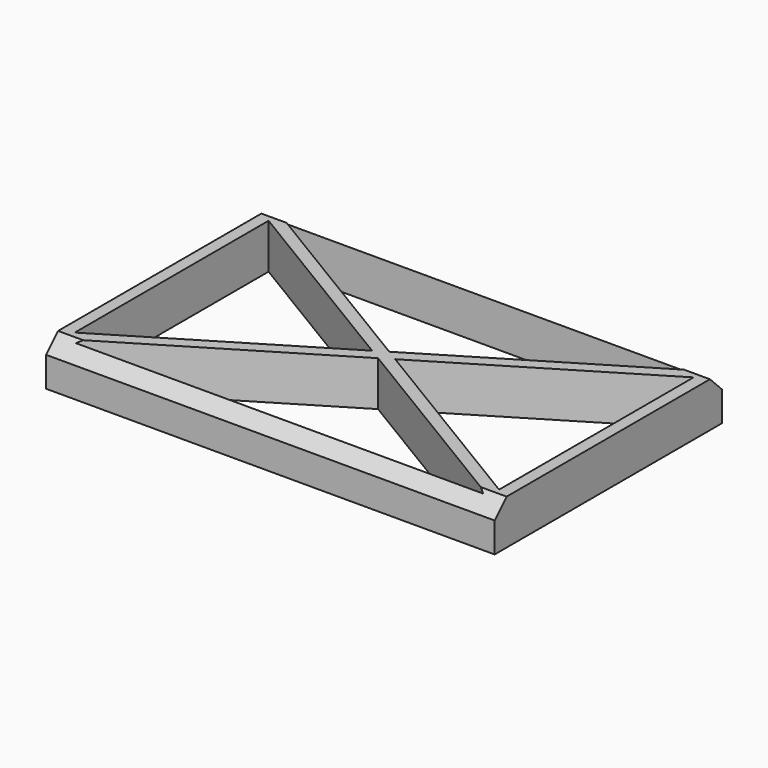
from build123d import *

# Parameters (mm, degrees)
F0_W        = 38.1
F0_H        = 24.13
F1_DEPTH    = 3.81
F2_T1_DEPTH = 44.6320747894


# Not quite as in the source:
# - a fillet or chamfer that OpenCascade refuses, or shapes differently, is made with other operations: its cross-section is extruded or revolved along the edge and cut away or added


with BuildPart() as f1:
    # F0 (on Top) → F1 (new body)
    with BuildSketch(Plane.XY):
        Rectangle(F0_W, F0_H)
        Polygon((-0.029270627, -0.5935558801), (17.272, -11.049), (-17.330541254, -11.049), align=None, mode=Mode.SUBTRACT)
        Polygon((-18.034, -10.287), (-18.034, 10.287), (-1.0114642857, 0), align=None, mode=Mode.SUBTRACT)
        Polygon((-17.330541254, 11.049), (17.272, 11.049), (-0.029270627, 0.5935558801), align=None, mode=Mode.SUBTRACT)
        Polygon((0.9529230317, 0), (18.034, 10.3223774485), (18.034, -10.3223774485), align=None, mode=Mode.SUBTRACT)
    extrude(amount=F1_DEPTH)

    # F2: chamfer of 1.27 on 2 edges, made by hand

    # F2_s2 → F2_t1 (cut)
    with BuildSketch(Plane.YZ.offset(-22.3160373947)):
        Polygon((-12.065, 2.54), (-10.795, 3.81), (-12.065, 3.81), align=None)
        Polygon((12.065, 2.54), (10.795, 3.81), (12.065, 3.81), align=None)
    extrude(amount=F2_T1_DEPTH, mode=Mode.SUBTRACT)


solid = f1.part
